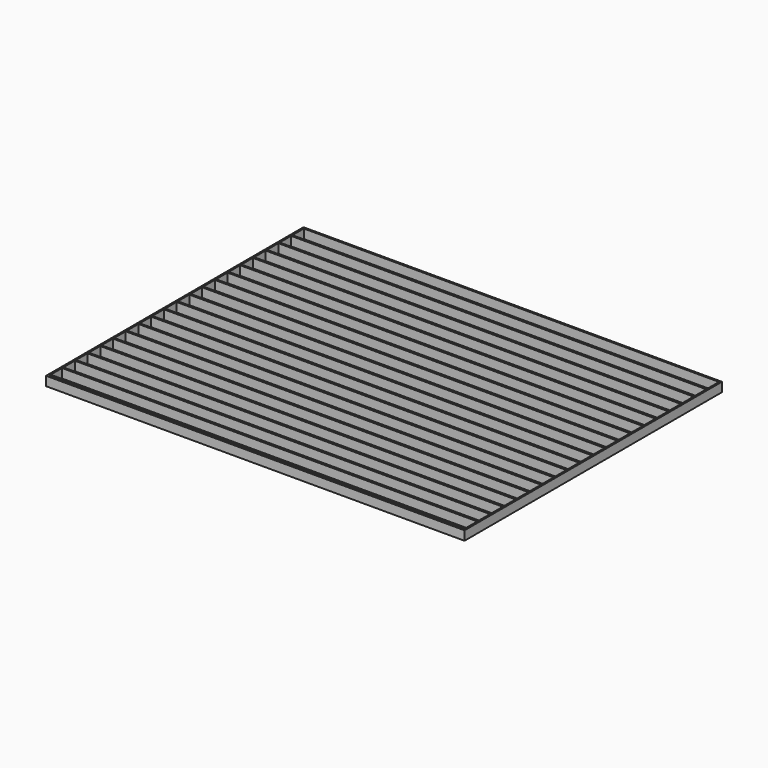
from build123d import *

# Parameters (mm, degrees)
F0_W     = 10693.2984
F0_H     = 8222.5896
F0_W_2   = 10611.0024
F0_H_2   = 41.148
F1_DEPTH = 234.95


with BuildPart() as f1:
    # F0 (on Top) → F1 (new body)
    with BuildSketch(Plane.XY):
        Rectangle(F0_W, F0_H)
        Polygon((5305.5012, -4057.8532), (5305.5012, -4070.1468), (-5305.5012, -4070.1468), (-5305.5012, -4057.8532), (-5305.5012, -4016.7052), (-5305.5012, -3651.4532), (-5305.5012, -3610.3052), (-5305.5012, -3245.0532), (-5305.5012, -3203.9052), (-5305.5012, -2838.6532), (-5305.5012, -2797.5052), (-5305.5012, -2432.2532), (-5305.5012, -2391.1052), (-5305.5012, -2025.8532), (-5305.5012, -1984.7052), (-5305.5012, -1619.4532), (-5305.5012, -1578.3052), (-5305.5012, -1213.0532), (-5305.5012, -1171.9052), (-5305.5012, -806.6532), (-5305.5012, -765.5052), (-5305.5012, -400.2532), (-5305.5012, -359.1052), (-5305.5012, 6.1468), (-5305.5012, 47.2948), (-5305.5012, 412.5468), (-5305.5012, 453.6948), (-5305.5012, 818.9468), (-5305.5012, 860.0948), (-5305.5012, 1225.3468), (-5305.5012, 1266.4948), (-5305.5012, 1631.7468), (-5305.5012, 1672.8948), (-5305.5012, 2038.1468), (-5305.5012, 2079.2948), (-5305.5012, 2444.5468), (-5305.5012, 2485.6948), (-5305.5012, 2850.9468), (-5305.5012, 2892.0948), (-5305.5012, 3257.3468), (-5305.5012, 3298.4948), (-5305.5012, 3663.7468), (-5305.5012, 3704.8948), (-5305.5012, 4070.1468), (5305.5012, 4070.1468), (5305.5012, 3704.8948), (5305.5012, 3663.7468), (5305.5012, 3298.4948), (5305.5012, 3257.3468), (5305.5012, 2892.0948), (5305.5012, 2850.9468), (5305.5012, 2485.6948), (5305.5012, 2444.5468), (5305.5012, 2079.2948), (5305.5012, 2038.1468), (5305.5012, 1672.8948), (5305.5012, 1631.7468), (5305.5012, 1266.4948), (5305.5012, 1225.3468), (5305.5012, 860.0948), (5305.5012, 818.9468), (5305.5012, 453.6948), (5305.5012, 412.5468), (5305.5012, 47.2948), (5305.5012, 6.1468), (5305.5012, -359.1052), (5305.5012, -400.2532), (5305.5012, -765.5052), (5305.5012, -806.6532), (5305.5012, -1171.9052), (5305.5012, -1213.0532), (5305.5012, -1578.3052), (5305.5012, -1619.4532), (5305.5012, -1984.7052), (5305.5012, -2025.8532), (5305.5012, -2391.1052), (5305.5012, -2432.2532), (5305.5012, -2797.5052), (5305.5012, -2838.6532), (5305.5012, -3203.9052), (5305.5012, -3245.0532), (5305.5012, -3610.3052), (5305.5012, -3651.4532), (5305.5012, -4016.7052), align=None, mode=Mode.SUBTRACT)
        with Locations((0, 3684.3208)):
            Rectangle(F0_W_2, F0_H_2)
        with Locations((0, 3277.9208)):
            Rectangle(F0_W_2, F0_H_2)
        with Locations((0, 2871.5208)):
            Rectangle(F0_W_2, F0_H_2)
        with Locations((0, 2465.1208)):
            Rectangle(F0_W_2, F0_H_2)
        with Locations((0, 2058.7208)):
            Rectangle(F0_W_2, F0_H_2)
        with Locations((0, 1652.3208)):
            Rectangle(F0_W_2, F0_H_2)
        with Locations((0, 1245.9208)):
            Rectangle(F0_W_2, F0_H_2)
        with Locations((0, 839.5208)):
            Rectangle(F0_W_2, F0_H_2)
        with Locations((0, 433.1208)):
            Rectangle(F0_W_2, F0_H_2)
        with Locations((0, 26.7208)):
            Rectangle(F0_W_2, F0_H_2)
        with Locations((0, -379.6792)):
            Rectangle(F0_W_2, F0_H_2)
        with Locations((0, -786.0792)):
            Rectangle(F0_W_2, F0_H_2)
        with Locations((0, -1192.4792)):
            Rectangle(F0_W_2, F0_H_2)
        with Locations((0, -1598.8792)):
            Rectangle(F0_W_2, F0_H_2)
        with Locations((0, -2005.2792)):
            Rectangle(F0_W_2, F0_H_2)
        with Locations((0, -2411.6792)):
            Rectangle(F0_W_2, F0_H_2)
        with Locations((0, -2818.0792)):
            Rectangle(F0_W_2, F0_H_2)
        with Locations((0, -3224.4792)):
            Rectangle(F0_W_2, F0_H_2)
        with Locations((0, -3630.8792)):
            Rectangle(F0_W_2, F0_H_2)
        with Locations((0, -4037.2792)):
            Rectangle(F0_W_2, F0_H_2)
    extrude(amount=F1_DEPTH)


solid = f1.part
